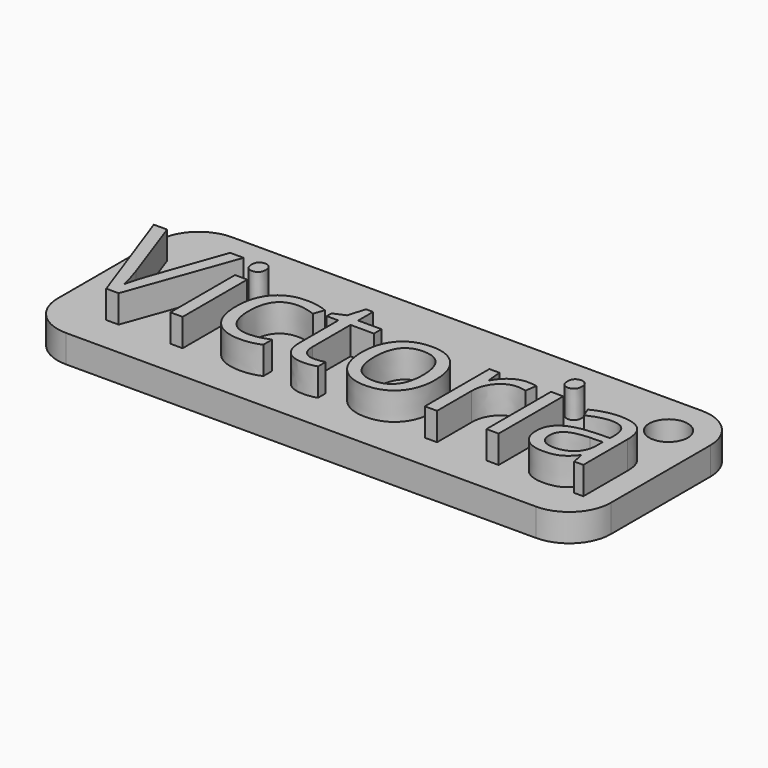
from build123d import *

# Parameters (mm, degrees)
F0_W         = 40
F0_H         = 15
F1_DEPTH     = 2
F2_TEXT_SIZE = 10.911701364
F3_DEPTH     = 2
F4_R         = 3
F6_R         = 1.3938059009
F7_DEPTH     = 2.001


# Not quite as in the source:
# - Text() gives the source's letters only with a copy of the font that has no kerning and outlines rounded to 1/6400 em; it was checked with that copy


with BuildPart() as f1:
    # F0 (on Top) → F1 (new body)
    with BuildSketch(Plane.XY):
        Rectangle(F0_W, F0_H)
    extrude(amount=F1_DEPTH)

    # F2 (on face) → F3 (join)
    with BuildSketch(Plane.XY.offset(2)):
        with Locations((-19, -4.84838001)):
            Text('Victoria', F2_TEXT_SIZE, font='Open Sans', text_align=(TextAlign.LEFT, TextAlign.BOTTOM))
    extrude(amount=F3_DEPTH)

    # F4
    f4_edges = [f1.edges().sort_by_distance(p)[0] for p in [
        (20, -7.5, 1),
        (20, 7.5, 1),
        (-20, -7.5, 1),
        (-20, 7.5, 1),
    ]]
    fillet(f4_edges, radius=F4_R)

    # F6 (on face) → F7 (cut, through all)
    with BuildSketch(Plane.XY.offset(2)):
        with Locations((17.0321103652, 4.425273584)):
            Circle(F6_R)
    extrude(amount=-F7_DEPTH, mode=Mode.SUBTRACT)


solid = f1.part
